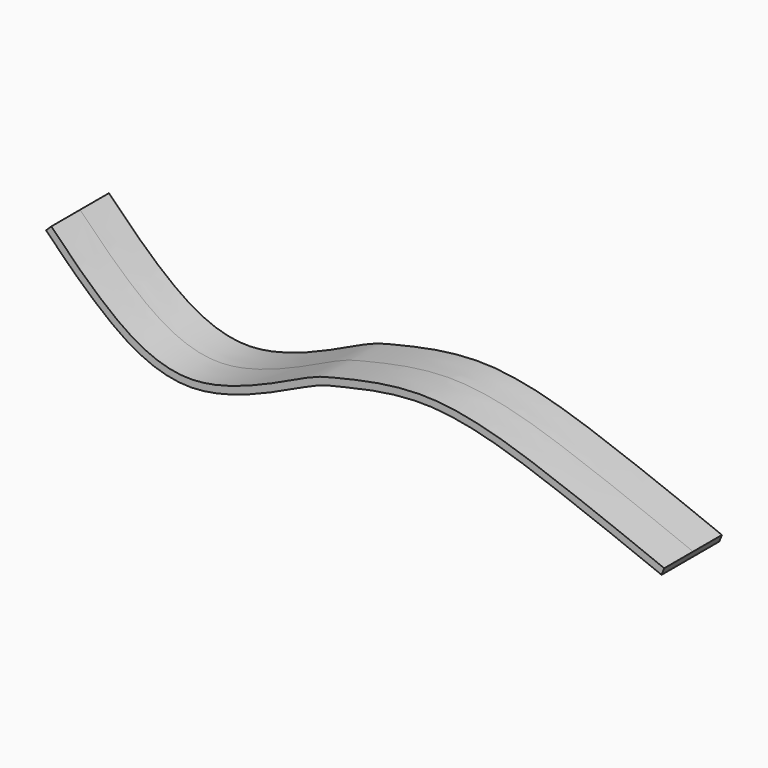
from build123d import *

# Parameters (mm, degrees)
F1_DEPTH = 12.7


# Not quite as in the source:
# - the dataset's text gives a spline's control points without its knots; the knots are read off the source's solid


with BuildPart() as f1:
    # F0 (on Front) → F1 (new body, symmetric)
    with BuildSketch(Plane.XZ):
        with BuildLine():
            add(Edge.make_bspline(
                [(0, 0), (5.8612335558, -6.0081148845), (18.3752479061, -18.835727906), (48.6654628653, -39.4932987315), (90.7530364795, -16.3272004333), (100.2814212382, -14.4870542481), (133.9403129455, -5.8103101016), (177.0386623069, -20.2782140016), (203.1498632313, -30.6887883047), (215.9, -35.7722866313)],
                knots=[0, 0, 0, 0, 0.129200241, 0.2758487022, 0.4410783086, 0.5233117279, 0.6646184967, 0.8362327321, 1, 1, 1, 1], degree=3))
            Line((0, 0), (-1.8181378704, -1.7736895682))
            add(Edge.make_bspline(
                [(-1.8181378704, -1.7736895682), (-0.4004659897, -3.2268880198), (2.4431142587, -6.1417829598), (6.8524053688, -10.5397610564), (10.7452755589, -14.2238690349), (14.0488962473, -17.1803558766), (16.2049401321, -19.0314128088), (17.9909210379, -20.5139707911), (19.8270649964, -21.9999559385), (22.2173956321, -23.8441638172), (25.2463744879, -25.9812516301), (28.4448239666, -27.9859413981), (31.822064763, -29.800697673), (35.386785102, -31.3660245692), (39.1456242468, -32.6202945152), (43.1015831462, -33.5005010422), (46.5604299892, -33.8694850047), (49.4218512492, -33.9167847472), (52.3425650521, -33.7869733676), (56.0409974594, -33.3140712632), (60.5186857591, -32.3465436646), (64.9836248523, -31.0633291737), (70.8500377765, -29.0399456974), (76.4748344801, -26.7059871293), (81.6189172058, -24.3744110822), (85.1730897504, -22.7052323037), (88.3552510159, -21.1961987948), (91.0972845141, -19.9257389393), (93.2887984197, -18.9941161488), (95.0891241303, -18.328556452), (96.6943622555, -17.8301427153), (98.0469088091, -17.4773372304), (99.2348494878, -17.1912683069), (100.197658958, -16.9654717597), (101.2546580452, -16.7179356412), (102.7954830873, -16.3504470242), (104.9344979714, -15.838506122), (107.8186019956, -15.175008387), (110.9802371747, -14.5008751611), (115.5133801016, -13.638792825), (120.4408484671, -12.9087974948), (125.5919935924, -12.463994437), (129.5259656126, -12.3090764437), (133.478060473, -12.3745703184), (137.4668709198, -12.6718476795), (141.4854505796, -13.175598953), (146.8725262766, -14.0979489105), (153.6404353633, -15.6692951637), (161.751337364, -18.0572248428), (169.7870128362, -20.7779992509), (177.689922634, -23.6529231388), (185.385108931, -26.529489533), (192.9176973961, -29.4196277885), (200.3292495735, -32.3175899877), (207.6621539732, -35.2222962334), (212.5263337706, -37.1616414275), (214.9593094143, -38.1316724035)],
                knots=[0, 0, 0, 0, 0.03125, 0.0625, 0.09375, 0.109375, 0.125, 0.1328125, 0.140625, 0.15625, 0.171875, 0.1875, 0.203125, 0.21875, 0.234375, 0.25, 0.265625, 0.2734375, 0.28125, 0.296875, 0.3125, 0.328125, 0.34375, 0.375, 0.390625, 0.40625, 0.421875, 0.4375, 0.453125, 0.46875, 0.484375, 0.5, 0.5078125, 0.515625, 0.5234375, 0.53125, 0.546875, 0.5625, 0.578125, 0.59375, 0.625, 0.640625, 0.65625, 0.671875, 0.6875, 0.703125, 0.71875, 0.75, 0.78125, 0.8125, 0.84375, 0.875, 0.90625, 0.9375, 0.96875, 1, 1, 1, 1], degree=3))
            Line((214.9593094143, -38.1316724035), (215.9, -35.7722866313))
        make_face()
    extrude(amount=F1_DEPTH, both=True)


solid = f1.part
